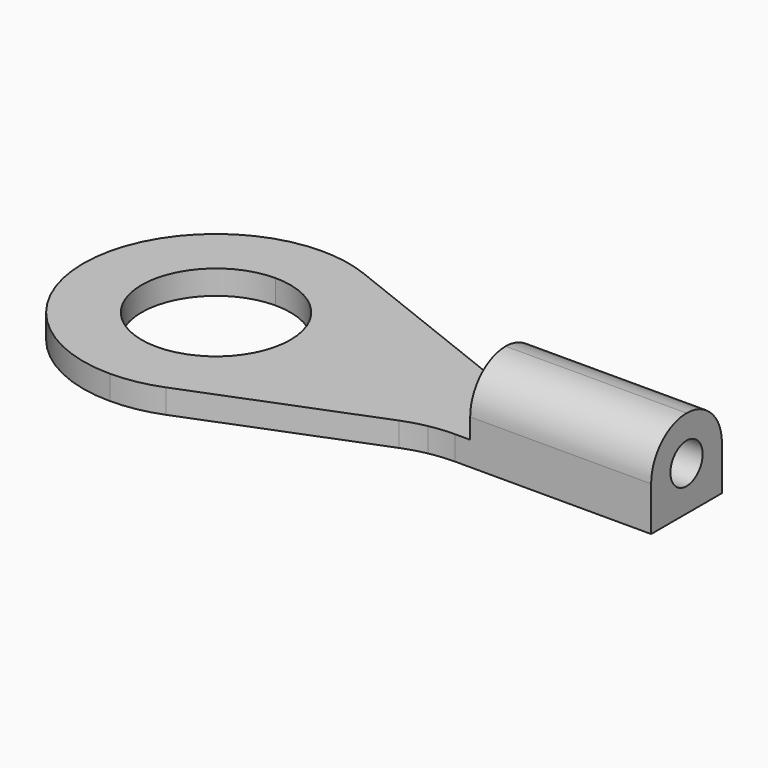
from build123d import *

# Parameters (mm, degrees)
F0_W     = 4.5
F0_H     = 1.1
F1_DEPTH = 0.6
F2_W     = 4.5
F2_H     = 2.2
F3_DEPTH = 1.6
F4_R     = 1.09999
F5_R     = 0.5
F6_DEPTH = 25


# Not quite as in the source:
# - a fillet or chamfer is up to 0.001 mm smaller than in the source, because OpenCascade refuses the exact size


with BuildPart() as f1:
    # F0 (on Top) → F1 (new body)
    with BuildSketch(Plane.XY):
        with Locations((12.75, 2.75)):
            Rectangle(F0_W, F0_H)
        with Locations((12.75, 3.85)):
            Rectangle(F0_W, F0_H)
        with BuildLine():
            Line((10.1278736967, 2.2), (10.5, 2.2))
            Line((10.5, 2.2), (10.5, 3.3))
            Line((10.5, 3.3), (9.5, 3.3))
            Line((9.5, 3.3), (9.5, 2.1397182935))
            ThreePointArc((9.5, 2.1397182935), (9.8124932664, 2.1848950035), (10.1278736967, 2.2))
        make_face()
        with BuildLine():
            Line((9.5, 3.3), (10.5, 3.3))
            Line((10.5, 3.3), (10.5, 4.4))
            Line((10.5, 4.4), (10.1278736967, 4.4))
            ThreePointArc((10.1278736967, 4.4), (9.8124932664, 4.4151049965), (9.5, 4.4602817065))
            Line((9.5, 4.4602817065), (9.5, 3.3))
        make_face()
        with BuildLine():
            Line((9.5, 2.1397182935), (9.5, 3.3))
            Line((9.5, 3.3), (9.5, 4.4602817065))
            ThreePointArc((9.5, 4.4602817065), (9.2040660975, 4.5319438894), (8.9159970588, 4.6305774135))
            Line((8.9159970588, 4.6305774135), (4.5118766379, 6.3694225865))
            ThreePointArc((4.5118766379, 6.3694225865), (3.9168085053, 6.5418431899), (3.3, 6.6))
            Line((3.3, 6.6), (3.3, 5.15))
            ThreePointArc((3.3, 5.15), (4.6081475452, 4.6081475452), (5.15, 3.3))
            ThreePointArc((5.15, 3.3), (4.6081475452, 1.9918524548), (3.3, 1.45))
            Line((3.3, 1.45), (3.3, 0))
            ThreePointArc((3.3, 0), (3.9168085053, 0.0581568101), (4.5118766379, 0.2305774135))
            Line((4.5118766379, 0.2305774135), (8.9159970588, 1.9694225865))
            ThreePointArc((8.9159970588, 1.9694225865), (9.2040660975, 2.0680561106), (9.5, 2.1397182935))
        make_face()
        with BuildLine():
            ThreePointArc((0, 3.3), (0.9665476221, 0.9665476221), (3.3, 0))
            Line((3.3, 0), (3.3, 1.45))
            ThreePointArc((3.3, 1.45), (1.45, 3.3), (3.3, 5.15))
            Line((3.3, 5.15), (3.3, 6.6))
            ThreePointArc((3.3, 6.6), (0.9665476221, 5.6334523779), (0, 3.3))
        make_face()
    extrude(amount=F1_DEPTH)

    # F2 (on face) → F3 (join)
    with BuildSketch(Plane.XY.offset(0.6)):
        with Locations((12.75, 3.3)):
            Rectangle(F2_W, F2_H)
    extrude(amount=F3_DEPTH)

    # F4 (radius 1.1 in the source; OpenCascade refuses exactly that, so slightly less here)
    f4_edges = [f1.edges().sort_by_distance(p)[0] for p in [
        (12.75, 2.2, 2.2),
        (12.75, 4.4, 2.2),
    ]]
    fillet(f4_edges, radius=F4_R)

    # F5 (on face) → F6 (cut)
    with BuildSketch(Plane.YZ.offset(15)):
        with Locations((3.3, 1.1)):
            Circle(F5_R)
    extrude(amount=-F6_DEPTH, mode=Mode.SUBTRACT)


solid = f1.part
